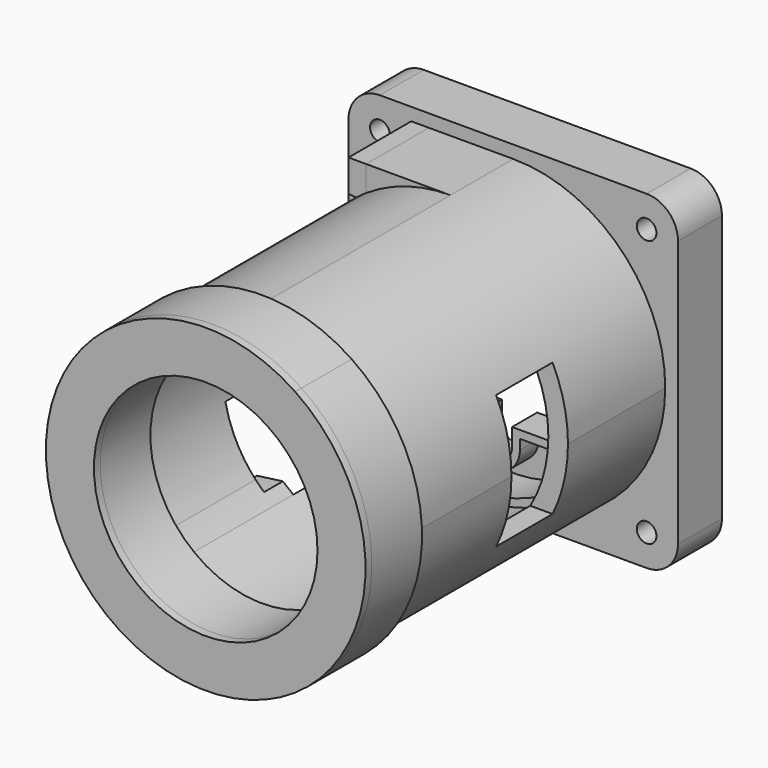
from build123d import *

# Parameters (mm, degrees)
F0_R      = 1.25
F1_DEPTH  = 4
F2_DEPTH  = 2
F3_R      = 1.25
F4_DEPTH  = 1
F5_DEPTH  = 4
F7_DEPTH  = 48
F8_DEPTH  = 48
F9_DEPTH  = 10
F10_DEPTH = 10
F6_R      = 15.875
F11_DEPTH = 5
F13_W     = 3
F13_H     = 10
F14_DEPTH = 20
F14_TAPER = 5
F12_W     = 9
F12_H     = 17
F15_DEPTH = 25
F16_R     = 14.25
F17_DEPTH = 1
F18_DEPTH = 8
F19_R     = 1.25
F20_DEPTH = 8


with BuildPart() as f1:
    # F0 (on Front) → F1 (new body)
    with BuildSketch(Plane.XZ):
        with BuildLine():
            ThreePointArc((-13, 17), (-13.2257453718, 18.3247648854), (-13.8775010008, 19.5))
            Line((-13.8775010008, 19.5), (-17, 19.5))
            ThreePointArc((-17, 19.5), (-18.767766953, 18.767766953), (-19.5, 17))
            Line((-19.5, 17), (-19.5, 13.8775010008))
            ThreePointArc((-19.5, 13.8775010008), (-15.2679491924, 13.3944487245), (-13, 17))
        make_face()
        with Locations((-17, 17)):
            Circle(F0_R, mode=Mode.SUBTRACT)
        with BuildLine():
            ThreePointArc((19.5, 17), (18.767766953, 18.767766953), (17, 19.5))
            Line((17, 19.5), (13.8775010008, 19.5))
            ThreePointArc((13.8775010008, 19.5), (14.1715728753, 14.1715728753), (19.5, 13.8775010008))
            Line((19.5, 13.8775010008), (19.5, 17))
        make_face()
        with Locations((17, 17)):
            Circle(F0_R, mode=Mode.SUBTRACT)
        with BuildLine():
            Line((19.5, -17), (19.5, -14.5))
            ThreePointArc((19.5, -14.5), (14.5, -14.5), (14.5, -19.5))
            Line((14.5, -19.5), (17, -19.5))
            ThreePointArc((17, -19.5), (18.767766953, -18.767766953), (19.5, -17))
        make_face()
        with Locations((17, -17)):
            Circle(F0_R, mode=Mode.SUBTRACT)
        with BuildLine():
            ThreePointArc((-13, -17), (-15.2679491924, -13.3944487245), (-19.5, -13.8775010008))
            Line((-19.5, -13.8775010008), (-19.5, -17))
            ThreePointArc((-19.5, -17), (-18.767766953, -18.767766953), (-17, -19.5))
            Line((-17, -19.5), (-13.8775010008, -19.5))
            ThreePointArc((-13.8775010008, -19.5), (-13.2257453718, -18.3247648854), (-13, -17))
        make_face()
        with Locations((-17, -17)):
            Circle(F0_R, mode=Mode.SUBTRACT)
        with BuildLine():
            Line((-19.5, -13.8775010008), (-19.5, 13.8775010008))
            ThreePointArc((-19.5, 13.8775010008), (-20.6055512755, 15.2679491924), (-21, 17))
            Line((-21, 17), (-21, -17))
            ThreePointArc((-21, -17), (-20.6055512755, -15.2679491924), (-19.5, -13.8775010008))
        make_face()
        with BuildLine():
            ThreePointArc((21, 17), (20.6055512755, 15.2679491924), (19.5, 13.8775010008))
            Line((19.5, 13.8775010008), (19.5, -14.5))
            ThreePointArc((19.5, -14.5), (20.2664074122, -15.6470097496), (20.5355339059, -17))
            ThreePointArc((20.5355339059, -17), (18.3529902504, -20.2664074122), (14.5, -19.5))
            Line((14.5, -19.5), (-13.8775010008, -19.5))
            ThreePointArc((-13.8775010008, -19.5), (-15.2679491924, -20.6055512755), (-17, -21))
            Line((-17, -21), (17, -21))
            ThreePointArc((17, -21), (19.8284271247, -19.8284271247), (21, -17))
            Line((21, -17), (21, 17))
        make_face()
        with BuildLine():
            Line((-17, 19.5), (-13.8775010008, 19.5))
            ThreePointArc((-13.8775010008, 19.5), (-15.2679491924, 20.6055512755), (-17, 21))
            ThreePointArc((-17, 21), (-19.8284271247, 19.8284271247), (-21, 17))
            ThreePointArc((-21, 17), (-20.6055512755, 15.2679491924), (-19.5, 13.8775010008))
            Line((-19.5, 13.8775010008), (-19.5, 17))
            ThreePointArc((-19.5, 17), (-18.767766953, 18.767766953), (-17, 19.5))
        make_face()
        with BuildLine():
            Line((-13.8775010008, 19.5), (13.8775010008, 19.5))
            ThreePointArc((13.8775010008, 19.5), (15.2679491924, 20.6055512755), (17, 21))
            Line((17, 21), (-17, 21))
            ThreePointArc((-17, 21), (-15.2679491924, 20.6055512755), (-13.8775010008, 19.5))
        make_face()
        with BuildLine():
            Line((13.8775010008, 19.5), (17, 19.5))
            ThreePointArc((17, 19.5), (18.767766953, 18.767766953), (19.5, 17))
            Line((19.5, 17), (19.5, 13.8775010008))
            ThreePointArc((19.5, 13.8775010008), (20.6055512755, 15.2679491924), (21, 17))
            ThreePointArc((21, 17), (19.8284271247, 19.8284271247), (17, 21))
            ThreePointArc((17, 21), (15.2679491924, 20.6055512755), (13.8775010008, 19.5))
        make_face()
        with BuildLine():
            ThreePointArc((20.5355339059, -17), (20.2664074122, -15.6470097496), (19.5, -14.5))
            Line((19.5, -14.5), (19.5, -17))
            ThreePointArc((19.5, -17), (18.767766953, -18.767766953), (17, -19.5))
            Line((17, -19.5), (14.5, -19.5))
            ThreePointArc((14.5, -19.5), (18.3529902504, -20.2664074122), (20.5355339059, -17))
        make_face()
        with BuildLine():
            Line((-19.5, -17), (-19.5, -13.8775010008))
            ThreePointArc((-19.5, -13.8775010008), (-20.6055512755, -15.2679491924), (-21, -17))
            ThreePointArc((-21, -17), (-19.8284271247, -19.8284271247), (-17, -21))
            ThreePointArc((-17, -21), (-15.2679491924, -20.6055512755), (-13.8775010008, -19.5))
            Line((-13.8775010008, -19.5), (-17, -19.5))
            ThreePointArc((-17, -19.5), (-18.767766953, -18.767766953), (-19.5, -17))
        make_face()
    extrude(amount=F1_DEPTH)

    # F0 (on Front) → F2 (join)
    with BuildSketch(Plane.XZ):
        with BuildLine():
            Line((-13.8775010008, 19.5), (13.8775010008, 19.5))
            ThreePointArc((13.8775010008, 19.5), (15.2679491924, 20.6055512755), (17, 21))
            Line((17, 21), (-17, 21))
            ThreePointArc((-17, 21), (-15.2679491924, 20.6055512755), (-13.8775010008, 19.5))
        make_face()
        with BuildLine():
            Line((13.8775010008, 19.5), (17, 19.5))
            ThreePointArc((17, 19.5), (18.767766953, 18.767766953), (19.5, 17))
            Line((19.5, 17), (19.5, 13.8775010008))
            ThreePointArc((19.5, 13.8775010008), (20.6055512755, 15.2679491924), (21, 17))
            ThreePointArc((21, 17), (19.8284271247, 19.8284271247), (17, 21))
            ThreePointArc((17, 21), (15.2679491924, 20.6055512755), (13.8775010008, 19.5))
        make_face()
        with BuildLine():
            Line((-17, 19.5), (-13.8775010008, 19.5))
            ThreePointArc((-13.8775010008, 19.5), (-15.2679491924, 20.6055512755), (-17, 21))
            ThreePointArc((-17, 21), (-19.8284271247, 19.8284271247), (-21, 17))
            ThreePointArc((-21, 17), (-20.6055512755, 15.2679491924), (-19.5, 13.8775010008))
            Line((-19.5, 13.8775010008), (-19.5, 17))
            ThreePointArc((-19.5, 17), (-18.767766953, 18.767766953), (-17, 19.5))
        make_face()
        with BuildLine():
            Line((-19.5, -13.8775010008), (-19.5, 13.8775010008))
            ThreePointArc((-19.5, 13.8775010008), (-20.6055512755, 15.2679491924), (-21, 17))
            Line((-21, 17), (-21, -17))
            ThreePointArc((-21, -17), (-20.6055512755, -15.2679491924), (-19.5, -13.8775010008))
        make_face()
        with BuildLine():
            Line((-19.5, -17), (-19.5, -13.8775010008))
            ThreePointArc((-19.5, -13.8775010008), (-20.6055512755, -15.2679491924), (-21, -17))
            ThreePointArc((-21, -17), (-19.8284271247, -19.8284271247), (-17, -21))
            ThreePointArc((-17, -21), (-15.2679491924, -20.6055512755), (-13.8775010008, -19.5))
            Line((-13.8775010008, -19.5), (-17, -19.5))
            ThreePointArc((-17, -19.5), (-18.767766953, -18.767766953), (-19.5, -17))
        make_face()
        with BuildLine():
            ThreePointArc((21, 17), (20.6055512755, 15.2679491924), (19.5, 13.8775010008))
            Line((19.5, 13.8775010008), (19.5, -14.5))
            ThreePointArc((19.5, -14.5), (20.2664074122, -15.6470097496), (20.5355339059, -17))
            ThreePointArc((20.5355339059, -17), (18.3529902504, -20.2664074122), (14.5, -19.5))
            Line((14.5, -19.5), (-13.8775010008, -19.5))
            ThreePointArc((-13.8775010008, -19.5), (-15.2679491924, -20.6055512755), (-17, -21))
            Line((-17, -21), (17, -21))
            ThreePointArc((17, -21), (19.8284271247, -19.8284271247), (21, -17))
            Line((21, -17), (21, 17))
        make_face()
        with BuildLine():
            ThreePointArc((20.5355339059, -17), (20.2664074122, -15.6470097496), (19.5, -14.5))
            Line((19.5, -14.5), (19.5, -17))
            ThreePointArc((19.5, -17), (18.767766953, -18.767766953), (17, -19.5))
            Line((17, -19.5), (14.5, -19.5))
            ThreePointArc((14.5, -19.5), (18.3529902504, -20.2664074122), (20.5355339059, -17))
        make_face()
    extrude(amount=-F2_DEPTH)

    # F3 (on face) → F4 (join)
    with BuildSketch(Plane.XZ.offset(4)):
        with BuildLine():
            Line((17, 21), (-17, 21))
            ThreePointArc((-17, 21), (-19.8284271247, 19.8284271247), (-21, 17))
            Line((-21, 17), (-21, -17))
            ThreePointArc((-21, -17), (-19.8284271247, -19.8284271247), (-17, -21))
            Line((-17, -21), (17, -21))
            ThreePointArc((17, -21), (19.8284271247, -19.8284271247), (21, -17))
            Line((21, -17), (21, 17))
            ThreePointArc((21, 17), (19.8284271247, 19.8284271247), (17, 21))
        make_face()
        with Locations((-17, -17)):
            Circle(F3_R, mode=Mode.SUBTRACT)
        with Locations((17, -17)):
            Circle(F3_R, mode=Mode.SUBTRACT)
        with Locations((-17, 17)):
            Circle(F3_R, mode=Mode.SUBTRACT)
        with BuildLine():
            ThreePointArc((-13.8775010008, -19.5), (-14.1715728753, -14.1715728753), (-19.5, -13.8775010008))
            Line((-19.5, -13.8775010008), (-19.5, 13.8775010008))
            ThreePointArc((-19.5, 13.8775010008), (-14.1715728753, 14.1715728753), (-13.8775010008, 19.5))
            Line((-13.8775010008, 19.5), (13.8775010008, 19.5))
            ThreePointArc((13.8775010008, 19.5), (14.1715728753, 14.1715728753), (19.5, 13.8775010008))
            Line((19.5, 13.8775010008), (19.5, -14.5))
            ThreePointArc((19.5, -14.5), (14.5, -14.5), (14.5, -19.5))
            Line((14.5, -19.5), (-13.8775010008, -19.5))
        make_face(mode=Mode.SUBTRACT)
        with Locations((17, 17)):
            Circle(F3_R, mode=Mode.SUBTRACT)
        with BuildLine():
            Line((-19.5, 13.8775010008), (-19.5, -13.8775010008))
            ThreePointArc((-19.5, -13.8775010008), (-14.1715728753, -14.1715728753), (-13.8775010008, -19.5))
            Line((-13.8775010008, -19.5), (14.5, -19.5))
            ThreePointArc((14.5, -19.5), (14.5, -14.5), (19.5, -14.5))
            Line((19.5, -14.5), (19.5, 13.8775010008))
            ThreePointArc((19.5, 13.8775010008), (14.1715728753, 14.1715728753), (13.8775010008, 19.5))
            Line((13.8775010008, 19.5), (-13.8775010008, 19.5))
            ThreePointArc((-13.8775010008, 19.5), (-14.1715728753, 14.1715728753), (-19.5, 13.8775010008))
        make_face()
        with BuildLine():
            ThreePointArc((3.25, -11), (0, -14.25), (-3.25, -11))
            Line((-3.25, -11), (-3.25, -9.75))
            Line((-3.25, -9.75), (-9.75, -9.75))
            Line((-9.75, -9.75), (-9.75, 9.75))
            Line((-9.75, 9.75), (-3.25, 9.75))
            Line((-3.25, 9.75), (-3.25, 11))
            ThreePointArc((-3.25, 11), (0, 14.25), (3.25, 11))
            Line((3.25, 11), (3.25, 9.75))
            Line((3.25, 9.75), (9.75, 9.75))
            Line((9.75, 9.75), (9.75, -9.75))
            Line((9.75, -9.75), (3.25, -9.75))
            Line((3.25, -9.75), (3.25, -11))
        make_face(mode=Mode.SUBTRACT)
        with BuildLine():
            Line((-3.25, -9.75), (-3.25, -11))
            ThreePointArc((-3.25, -11), (0, -14.25), (3.25, -11))
            Line((3.25, -11), (3.25, -9.75))
            Line((3.25, -9.75), (9.75, -9.75))
            Line((9.75, -9.75), (9.75, 9.75))
            Line((9.75, 9.75), (3.25, 9.75))
            Line((3.25, 9.75), (3.25, 11))
            ThreePointArc((3.25, 11), (0, 14.25), (-3.25, 11))
            Line((-3.25, 11), (-3.25, 9.75))
            Line((-3.25, 9.75), (-9.75, 9.75))
            Line((-9.75, 9.75), (-9.75, -9.75))
            Line((-9.75, -9.75), (-3.25, -9.75))
        make_face()
        with BuildLine():
            Line((2.25, 8.75), (8.75, 8.75))
            Line((8.75, 8.75), (8.75, -8.75))
            Line((8.75, -8.75), (2.25, -8.75))
            Line((2.25, -8.75), (2.25, -11))
            ThreePointArc((2.25, -11), (0, -13.25), (-2.25, -11))
            Line((-2.25, -11), (-2.25, -8.75))
            Line((-2.25, -8.75), (-8.75, -8.75))
            Line((-8.75, -8.75), (-8.75, 8.75))
            Line((-8.75, 8.75), (-2.25, 8.75))
            Line((-2.25, 8.75), (-2.25, 11))
            ThreePointArc((-2.25, 11), (0, 13.25), (2.25, 11))
            Line((2.25, 11), (2.25, 8.75))
        make_face(mode=Mode.SUBTRACT)
    extrude(amount=F4_DEPTH)

    # F3 (on face) → F5 (join)
    with BuildSketch(Plane.XZ.offset(4)):
        with BuildLine():
            Line((-3.25, -9.75), (-3.25, -11))
            ThreePointArc((-3.25, -11), (0, -14.25), (3.25, -11))
            Line((3.25, -11), (3.25, -9.75))
            Line((3.25, -9.75), (9.75, -9.75))
            Line((9.75, -9.75), (9.75, 9.75))
            Line((9.75, 9.75), (3.25, 9.75))
            Line((3.25, 9.75), (3.25, 11))
            ThreePointArc((3.25, 11), (0, 14.25), (-3.25, 11))
            Line((-3.25, 11), (-3.25, 9.75))
            Line((-3.25, 9.75), (-9.75, 9.75))
            Line((-9.75, 9.75), (-9.75, -9.75))
            Line((-9.75, -9.75), (-3.25, -9.75))
        make_face()
        with BuildLine():
            Line((2.25, 8.75), (8.75, 8.75))
            Line((8.75, 8.75), (8.75, -8.75))
            Line((8.75, -8.75), (2.25, -8.75))
            Line((2.25, -8.75), (2.25, -11))
            ThreePointArc((2.25, -11), (0, -13.25), (-2.25, -11))
            Line((-2.25, -11), (-2.25, -8.75))
            Line((-2.25, -8.75), (-8.75, -8.75))
            Line((-8.75, -8.75), (-8.75, 8.75))
            Line((-8.75, 8.75), (-2.25, 8.75))
            Line((-2.25, 8.75), (-2.25, 11))
            ThreePointArc((-2.25, 11), (0, 13.25), (2.25, 11))
            Line((2.25, 11), (2.25, 8.75))
        make_face(mode=Mode.SUBTRACT)
    extrude(amount=F5_DEPTH)

    # F6 (on face) → F11 (join)
    with BuildSketch(Plane.XZ.offset(5)):
        with BuildLine():
            ThreePointArc((16.875, 0), (7.1888585673, 15.2671522394), (-10.75, 13.0078101539))
            ThreePointArc((-10.75, 13.0078101539), (-11.9280934404, 11.9367588514), (-13, 10.7594435265))
            ThreePointArc((-13, 10.7594435265), (-16.875, 0), (-13, -10.7594435265))
            ThreePointArc((-13, -10.7594435265), (-11.9280934404, -11.9367588514), (-10.75, -13.0078101539))
            ThreePointArc((-10.75, -13.0078101539), (7.1888585673, -15.2671522394), (16.875, 0))
        make_face()
        Circle(F6_R, mode=Mode.SUBTRACT)
    extrude(amount=F11_DEPTH)


with BuildPart() as f7:
    # F6 (on face) → F7 (new body)
    with BuildSketch(Plane.XZ.offset(5)):
        with BuildLine():
            ThreePointArc((0, -19.375), (13.7001938855, -13.7001938855), (19.375, 0))
            ThreePointArc((19.375, 0), (13.7001938855, 13.7001938855), (0, 19.375))
            ThreePointArc((0, 19.375), (-5.6161114512, 18.5431905876), (-10.75, 16.119184998))
            Line((-10.75, 16.119184998), (-10.75, 13.0078101539))
            ThreePointArc((-10.75, 13.0078101539), (7.1888585673, 15.2671522394), (16.875, 0))
            ThreePointArc((16.875, 0), (7.1888585673, -15.2671522394), (-10.75, -13.0078101539))
            Line((-10.75, -13.0078101539), (-10.75, -16.119184998))
            ThreePointArc((-10.75, -16.119184998), (-5.6161114512, -18.5431905876), (0, -19.375))
        make_face()
    extrude(amount=F7_DEPTH)

    # F6 (on face) → F9 (join)
    with BuildSketch(Plane.XZ.offset(5)):
        with BuildLine():
            Line((-10.75, -19.375), (0, -19.375))
            ThreePointArc((0, -19.375), (-5.6161114512, -18.5431905876), (-10.75, -16.119184998))
            Line((-10.75, -16.119184998), (-10.75, -19.375))
        make_face()
        with BuildLine():
            ThreePointArc((-10.75, 16.119184998), (-5.6161114512, 18.5431905876), (0, 19.375))
            Line((0, 19.375), (-10.75, 19.375))
            Line((-10.75, 19.375), (-10.75, 16.119184998))
        make_face()
    extrude(amount=F9_DEPTH)

    # F12 (on face) → F15 (cut)
    with BuildSketch(Plane.YZ.offset(21)):
        with Locations((-25, 0)):
            Rectangle(F12_W, F12_H)
    extrude(amount=-F15_DEPTH, mode=Mode.SUBTRACT)


with BuildPart() as f8:
    # F6 (on face) → F8 (new body)
    with BuildSketch(Plane.XZ.offset(5)):
        with BuildLine():
            Line((-13, 10.7594435265), (-13, 14.3663017162))
            ThreePointArc((-13, 14.3663017162), (-19.375, 0), (-13, -14.3663017162))
            Line((-13, -14.3663017162), (-13, -10.7594435265))
            ThreePointArc((-13, -10.7594435265), (-16.875, 0), (-13, 10.7594435265))
        make_face()
        with BuildLine():
            ThreePointArc((-13, -14.3663017162), (-11.9072992299, -15.2842026305), (-10.75, -16.119184998))
            Line((-10.75, -16.119184998), (-10.75, -13.0078101539))
            ThreePointArc((-10.75, -13.0078101539), (-11.9280934404, -11.9367588514), (-13, -10.7594435265))
            Line((-13, -10.7594435265), (-13, -14.3663017162))
        make_face()
        with BuildLine():
            Line((-10.75, 13.0078101539), (-10.75, 16.119184998))
            ThreePointArc((-10.75, 16.119184998), (-11.9072992299, 15.2842026305), (-13, 14.3663017162))
            Line((-13, 14.3663017162), (-13, 10.7594435265))
            ThreePointArc((-13, 10.7594435265), (-11.9280934404, 11.9367588514), (-10.75, 13.0078101539))
        make_face()
    extrude(amount=F8_DEPTH)

    # F6 (on face) → F10 (join)
    with BuildSketch(Plane.XZ.offset(5)):
        with BuildLine():
            Line((-10.75, -19.375), (-10.75, -16.119184998))
            ThreePointArc((-10.75, -16.119184998), (-11.9072992299, -15.2842026305), (-13, -14.3663017162))
            Line((-13, -14.3663017162), (-13, -19.375))
            Line((-13, -19.375), (-10.75, -19.375))
        make_face()
        with BuildLine():
            ThreePointArc((-13, 14.3663017162), (-11.9072992299, 15.2842026305), (-10.75, 16.119184998))
            Line((-10.75, 16.119184998), (-10.75, 19.375))
            Line((-10.75, 19.375), (-13, 19.375))
            Line((-13, 19.375), (-13, 14.3663017162))
        make_face()
    extrude(amount=F10_DEPTH)

    # F13 (on face) → F14 (cut)
    with BuildSketch(Plane(origin=(-21, 0, 0), x_dir=(0, -1, 0), z_dir=(-1, 0, 0))):
        Polygon((27.5, 16), (10, 16), (10, 0), (27.5, 0), (27.5, 15.3445341364), align=None)
        Polygon((27.5, 0), (10, 0), (10, -16), (10, -16.6554658636), (27.5, -16.6554658636), (27.5, -12.6554658636), (27.5, -2.6554658636), align=None)
        with Locations((29, -7.6554658636)):
            Rectangle(F13_W, F13_H)
    extrude(amount=-F14_DEPTH, taper=F14_TAPER, mode=Mode.SUBTRACT)


with BuildPart() as f17:
    # F16 (on face) → F17 (new body)
    with BuildSketch(Plane.XZ.offset(53)):
        with BuildLine():
            ThreePointArc((11.4038153521, -16.8847155858), (20.375, 0), (11.4038153521, 16.8847155858))
            ThreePointArc((11.4038153521, 16.8847155858), (-20.375, 0), (11.4038153521, -16.8847155858))
        make_face()
        with BuildLine():
            ThreePointArc((0, 19.375), (18.5431905876, -5.6161114512), (-10.75, -16.119184998))
            ThreePointArc((-10.75, -16.119184998), (-19.375, 0), (-10.75, 16.119184998))
            ThreePointArc((-10.75, 16.119184998), (-5.6161114512, 18.5431905876), (0, 19.375))
        make_face(mode=Mode.SUBTRACT)
        with BuildLine():
            ThreePointArc((-10.75, 13.0078101539), (-16.875, 0), (-10.75, -13.0078101539))
            ThreePointArc((-10.75, -13.0078101539), (16.875, 0), (-10.75, 13.0078101539))
        make_face()
        Circle(F16_R, mode=Mode.SUBTRACT)
        with BuildLine():
            Line((-10.75, -13.0078101539), (-10.75, -16.119184998))
            ThreePointArc((-10.75, -16.119184998), (18.5431905876, -5.6161114512), (0, 19.375))
            ThreePointArc((0, 19.375), (-5.6161114512, 18.5431905876), (-10.75, 16.119184998))
            Line((-10.75, 16.119184998), (-10.75, 13.0078101539))
            ThreePointArc((-10.75, 13.0078101539), (16.875, 0), (-10.75, -13.0078101539))
        make_face()
        with BuildLine():
            ThreePointArc((-10.75, 16.119184998), (-19.375, 0), (-10.75, -16.119184998))
            Line((-10.75, -16.119184998), (-10.75, -13.0078101539))
            ThreePointArc((-10.75, -13.0078101539), (-16.875, 0), (-10.75, 13.0078101539))
            Line((-10.75, 13.0078101539), (-10.75, 16.119184998))
        make_face()
    extrude(amount=F17_DEPTH)

    # F16 (on face) → F18 (join)
    with BuildSketch(Plane.XZ.offset(53)):
        with BuildLine():
            ThreePointArc((11.4038153521, -16.8847155858), (20.375, 0), (11.4038153521, 16.8847155858))
            ThreePointArc((11.4038153521, 16.8847155858), (-20.375, 0), (11.4038153521, -16.8847155858))
        make_face()
        with BuildLine():
            ThreePointArc((0, 19.375), (18.5431905876, -5.6161114512), (-10.75, -16.119184998))
            ThreePointArc((-10.75, -16.119184998), (-19.375, 0), (-10.75, 16.119184998))
            ThreePointArc((-10.75, 16.119184998), (-5.6161114512, 18.5431905876), (0, 19.375))
        make_face(mode=Mode.SUBTRACT)
        with BuildLine():
            ThreePointArc((-10.75, 13.0078101539), (-16.875, 0), (-10.75, -13.0078101539))
            ThreePointArc((-10.75, -13.0078101539), (16.875, 0), (-10.75, 13.0078101539))
        make_face()
        Circle(F16_R, mode=Mode.SUBTRACT)
    extrude(amount=-F18_DEPTH)


with BuildPart() as f20_tool:
    # F19 (on face) → F20 (new body)
    with BuildSketch(Plane(origin=(-13, 0, 0), x_dir=(0, -1, 0), z_dir=(-1, 0, 0))):
        with Locations((7.8499546541, -17.6652782777)):
            Circle(F19_R)
        with Locations((7.8499546541, 17.6652782777)):
            Circle(F19_R)
    extrude(amount=-F20_DEPTH)


with BuildPart() as f7_1:
    add(f7.part)

    # F20: cut by f20_tool
    add(f20_tool.part, mode=Mode.SUBTRACT)


with BuildPart() as f8_1:
    add(f8.part)

    # F20: cut by f20_tool
    add(f20_tool.part, mode=Mode.SUBTRACT)


solid = Compound([f1.part, f17.part, f7_1.part, f8_1.part])
